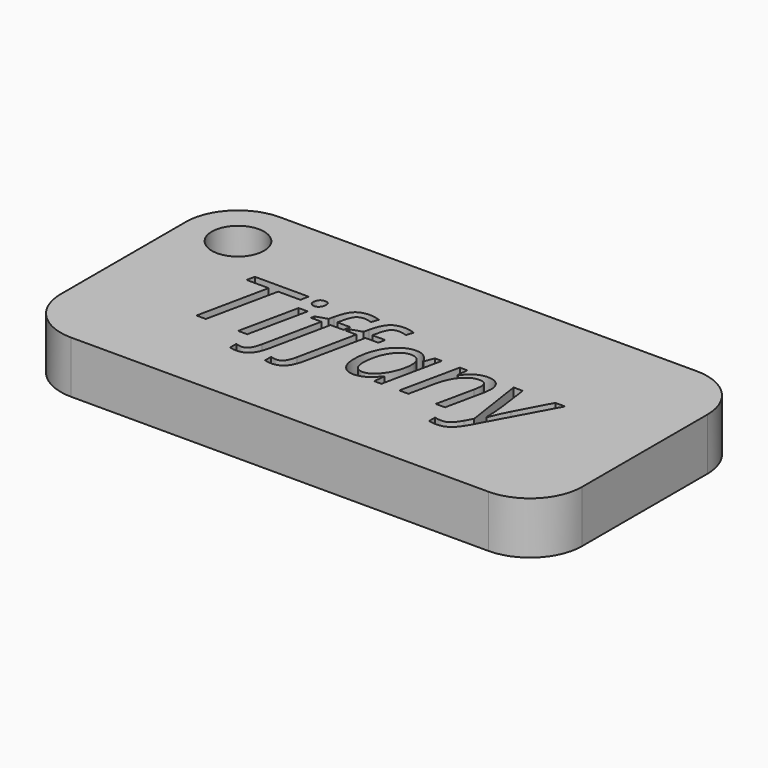
from build123d import *

# Parameters (mm, degrees)
F0_W         = 50.8
F0_H         = 25.4
F1_DEPTH     = 5.08
F2_TEXT_SIZE = 10.8667150237
F3_DEPTH     = 2.54
F4_R         = 5.08
F5_R         = 2.54
F6_DEPTH     = 25.4


# Not quite as in the source:
# - Text() gives the source's letters only with a copy of the font that has no kerning and outlines rounded to 1/6400 em; it was checked with that copy


with BuildPart() as f1:
    # F0 (on Top) → F1 (new body)
    with BuildSketch(Plane.XY):
        Rectangle(F0_W, F0_H)
    extrude(amount=F1_DEPTH)

    # F2 (on face) → F3 (cut)
    with BuildSketch(Plane.XY.offset(5.08)):
        with Locations((-16.8094498022, -3.9120174085)):
            Text('Tiffany', F2_TEXT_SIZE, font='Open Sans', font_style=FontStyle.ITALIC, text_align=(TextAlign.LEFT, TextAlign.BOTTOM))
    extrude(amount=-F3_DEPTH, mode=Mode.SUBTRACT)

    # F4
    f4_edges = [f1.edges().sort_by_distance(p)[0] for p in [
        (25.4, -12.7, 2.54),
        (25.4, 12.7, 2.54),
        (-25.4, 12.7, 2.54),
        (-25.4, -12.7, 2.54),
    ]]
    fillet(f4_edges, radius=F4_R)

    # F5 (on face) → F6 (cut)
    with BuildSketch(Plane.XY.offset(5.08)):
        with Locations((-20.32, 7.62)):
            Circle(F5_R)
    extrude(amount=-F6_DEPTH, mode=Mode.SUBTRACT)


solid = f1.part
